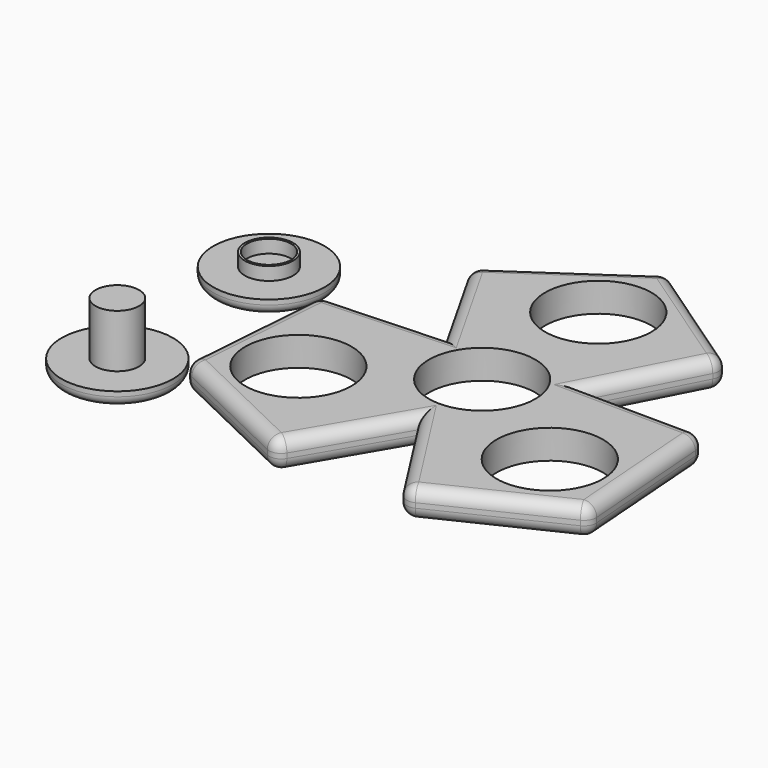
from build123d import *

# Parameters (mm, degrees)
F0_R      = 11
F1_DEPTH  = 6
F2_R      = 2.5
F3_R      = 11.5
F3_R_2    = 4.5
F6_DEPTH  = 3
F7_DEPTH  = 11
F8_DEPTH  = 3
F9_R      = 5
F9_R_2    = 4.55
F10_DEPTH = 3
F9_R_3    = 11.5
F11_DEPTH = 3
F12_DEPTH = 3
F14_R     = 11.5
F14_R_2   = 4.5
F15_DEPTH = 3
F16_DEPTH = 11
F17_R     = 2
F19_R     = 11.5
F19_R_2   = 5
F19_R_3   = 4.55
F20_DEPTH = 3
F21_DEPTH = 2.7
F22_R     = 2


# Not quite as in the source:
# - a feature names something its author has since deleted; it is built from what else it names
# - the program builds the solid bodies; features that only make, move or delete a surface that nothing else refers to are left out


with BuildPart() as f1:
    # F0 (on Top) → F1 (new body)
    with BuildSketch(Plane.XY):
        Polygon((25.8208357735, 30.5399207623), (0, 48.1595657766), (-26.6120665459, 30), (-14.2894191624, 8.25), (-39.3587650965, 7.0915393457), (-41.7074073978, -24.0797828883), (-12.6747288406, -38.0467256759), (0, -16.5), (13.5379293229, -37.631460108), (41.7074073978, -24.0797828883), (39.2867953865, 8.0467256759), (14.2894191624, 8.25), align=None)
        with Locations((-25.9807621135, -15)):
            Circle(F0_R, mode=Mode.SUBTRACT)
        Circle(F0_R, mode=Mode.SUBTRACT)
        with Locations((25.9807621135, -15)):
            Circle(F0_R, mode=Mode.SUBTRACT)
        with Locations((0, 30)):
            Circle(F0_R, mode=Mode.SUBTRACT)
    extrude(amount=F1_DEPTH)

    # F2
    f2_edges = [f1.edges().sort_by_distance(p)[0] for p in [
        (-13.306033, 39.079783, 0),
        (-13.306033, 39.079783, 6),
        (-20.450743, 19.125, 0),
        (-20.450743, 19.125, 6),
        (-26.824092, 7.67077, 0),
        (-26.824092, 7.67077, 6),
        (-40.533086, -8.494122, 0),
        (-40.533086, -8.494122, 6),
        (-27.191068, -31.063254, 0),
        (-27.191068, -31.063254, 6),
        (-6.337364, -27.273363, 0),
        (-6.337364, -27.273363, 6),
        (6.768965, -27.06573, 6),
        (6.768965, -27.06573, 0),
        (27.622668, -30.855621, 0),
        (27.622668, -30.855621, 6),
        (40.497101, -8.016529, 0),
        (40.497101, -8.016529, 6),
        (26.788107, 8.148363, 6),
        (20.055127, 19.39496, 6),
        (26.788107, 8.148363, 0),
        (20.055127, 19.39496, 0),
        (12.910418, 39.349743, 6),
        (12.910418, 39.349743, 0),
        (-39.358765, 7.091539, 3),
        (-26.612067, 30, 3),
        (0, 48.159566, 3),
        (25.820836, 30.539921, 3),
        (39.286795, 8.046726, 3),
        (41.707407, -24.079783, 3),
        (13.537929, -37.63146, 3),
        (-12.674729, -38.046726, 3),
        (-41.707407, -24.079783, 3),
    ]]
    fillet(f2_edges, radius=F2_R)


with BuildPart() as f6:
    # F3 (on Top) → F6 (new body)
    with BuildSketch(Plane.XY):
        with Locations((-56.0110025108, 44.7937771678)):
            Circle(F3_R)
        with Locations((-56.0110025108, 44.7937771678)):
            Circle(F3_R_2, mode=Mode.SUBTRACT)
    extrude(amount=-F6_DEPTH)


with BuildPart() as f7:
    # F3 (on Top) → F7 (new body)
    with BuildSketch(Plane.XY):
        with Locations((-56.0110025108, 44.7937771678)):
            Circle(F3_R_2)
    extrude(amount=F7_DEPTH)


with BuildPart() as f8:
    # F3 (on Top) → F8 (new body)
    with BuildSketch(Plane.XY):
        with Locations((-56.0110025108, 44.7937771678)):
            Circle(F3_R_2)
    extrude(amount=-F8_DEPTH)


with BuildPart() as f10:
    # F9 (on Top) → F10 (new body)
    with BuildSketch(Plane.XY):
        with Locations((-57.440303266, 13.5914236307)):
            Circle(F9_R)
        with Locations((-57.440303266, 13.5914236307)):
            Circle(F9_R_2, mode=Mode.SUBTRACT)
    extrude(amount=F10_DEPTH)

    # F9 (on Top) → F12 (join)
    with BuildSketch(Plane.XY):
        with Locations((-57.440303266, 13.5914236307)):
            Circle(F9_R_2)
    extrude(amount=-F12_DEPTH)


with BuildPart() as f11:
    # F9 (on Top) → F11 (new body)
    with BuildSketch(Plane.XY):
        with Locations((-57.440303266, 13.5914236307)):
            Circle(F9_R_3)
        with Locations((-57.440303266, 13.5914236307)):
            Circle(F9_R, mode=Mode.SUBTRACT)
    extrude(amount=-F11_DEPTH)


with BuildPart() as f15:
    # F14 (on Top) → F15 (new body)
    with BuildSketch(Plane.XY):
        with Locations((-57.7173270285, -22.1022814512)):
            Circle(F14_R)
        with Locations((-57.7173270285, -22.1022814512)):
            Circle(F14_R_2, mode=Mode.SUBTRACT)
        with Locations((-57.7173270285, -22.1022814512)):
            Circle(F14_R_2)
    extrude(amount=-F15_DEPTH)

    # F14 (on Top) → F16 (join)
    with BuildSketch(Plane.XY):
        with Locations((-57.7173270285, -22.1022814512)):
            Circle(F14_R_2)
    extrude(amount=F16_DEPTH)

    # F17
    f17_edges = [f15.edges().sort_by_distance(p)[0] for p in [
        (-69.217327, -22.102281, -3),
    ]]
    fillet(f17_edges, radius=F17_R)


with BuildPart() as f20:
    # F19 (on Top) → F20 (new body)
    with BuildSketch(Plane.XY):
        with Locations((-58.6504004896, 18.2378757745)):
            Circle(F19_R)
        with Locations((-58.6504004896, 18.2378757745)):
            Circle(F19_R_2, mode=Mode.SUBTRACT)
        with Locations((-58.6504004896, 18.2378757745)):
            Circle(F19_R_2)
        with Locations((-58.6504004896, 18.2378757745)):
            Circle(F19_R_3, mode=Mode.SUBTRACT)
        with Locations((-58.6504004896, 18.2378757745)):
            Circle(F19_R_3)
    extrude(amount=-F20_DEPTH)

    # F19 (on Top) → F21 (join)
    with BuildSketch(Plane.XY):
        with Locations((-58.6504004896, 18.2378757745)):
            Circle(F19_R_2)
        with Locations((-58.6504004896, 18.2378757745)):
            Circle(F19_R_3, mode=Mode.SUBTRACT)
    extrude(amount=F21_DEPTH)

    # F22
    f22_edges = [f20.edges().sort_by_distance(p)[0] for p in [
        (-70.1504, 18.237876, -3),
    ]]
    fillet(f22_edges, radius=F22_R)


solid = Compound([f1.part, f15.part, f20.part])
